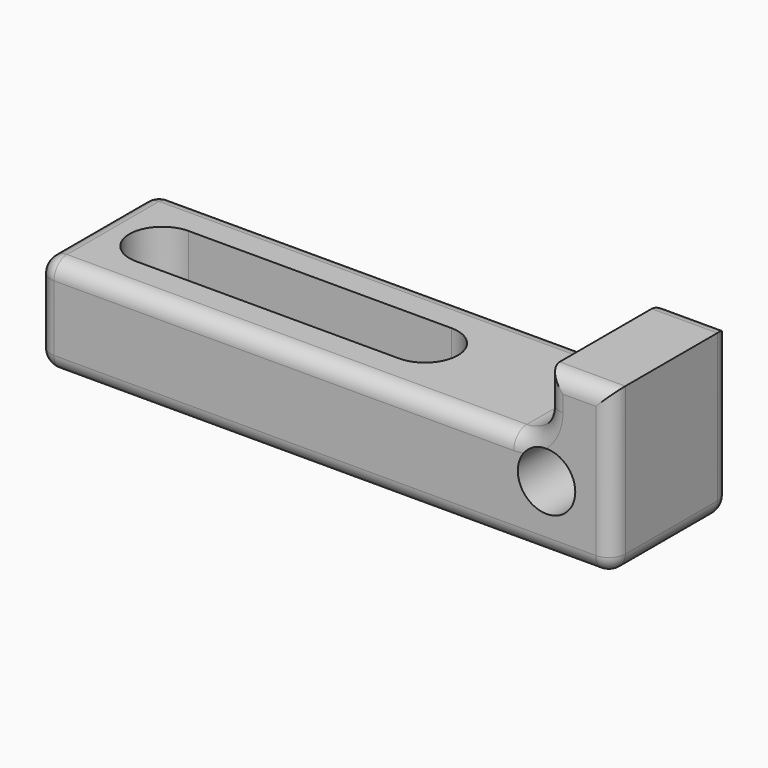
from build123d import *

# Parameters (mm, degrees)
F0_W         = 35
F0_H         = 9
F1_DEPTH     = 10
F2_R         = 1.75
F3_DEPTH     = 9.001
F5_DEPTH     = 6.001
F6_T1_DEPTH  = 28
F6_T3_DEPTH  = 7
F6_T5_DEPTH  = 9
F6_T7_DEPTH  = 33
F6_T9_DEPTH  = 4
F6_T11_DEPTH = 11.5
F6_T13_DEPTH = 4.5
F6_S17_W     = 1
F6_S17_H     = 1
F6_T18_DEPTH = 1
F6_S23_W     = 1
F6_S23_H     = 1
F6_T24_DEPTH = 1
F6_S29_W     = 1
F6_S29_H     = 1
F6_T30_DEPTH = 1
F6_S35_W     = 1
F6_S35_H     = 1
F6_T36_DEPTH = 1
F6_S41_W     = 1
F6_S41_H     = 1
F6_T42_DEPTH = 1
F6_S47_W     = 1
F6_S47_H     = 1
F6_T48_DEPTH = 1
F6_T52_ANGLE = 90
F6_T54_ANGLE = 90


# Not quite as in the source:
# - a fillet or chamfer that OpenCascade refuses, or shapes differently, is made with other operations: its cross-section is extruded or revolved along the edge and cut away or added


with BuildPart() as f1:
    # F0 (on Top) → F1 (new body)
    with BuildSketch(Plane.XY):
        Rectangle(F0_W, F0_H)
    extrude(amount=F1_DEPTH)

    # F2 (on face) → F3 (cut, through all)
    with BuildSketch(Plane.XZ.offset(4.5)):
        with BuildLine():
            Line((13.5, 10), (-17.5, 10))
            Line((-17.5, 10), (-17.5, 6))
            Line((-17.5, 6), (11.5, 6))
            ThreePointArc((11.5, 6), (12.9142135624, 6.5857864376), (13.5, 8))
            Line((13.5, 8), (13.5, 10))
        make_face()
        with Locations((13.5, 4)):
            Circle(F2_R)
    extrude(amount=-F3_DEPTH, mode=Mode.SUBTRACT)

    # F4 (on face) → F5 (cut, through all)
    with BuildSketch(Plane.XY.offset(6)):
        with BuildLine():
            ThreePointArc((-13.5, -2), (-12.0857864376, -1.4142135624), (-11.5, 0))
            ThreePointArc((-11.5, 0), (-12.0857864376, 1.4142135624), (-13.5, 2))
            ThreePointArc((-13.5, 2), (-15.5, 0), (-13.5, -2))
        make_face()
        with BuildLine():
            ThreePointArc((-13.5, 2), (-12.0857864376, 1.4142135624), (-11.5, 0))
            ThreePointArc((-11.5, 0), (-12.0857864376, -1.4142135624), (-13.5, -2))
            Line((-13.5, -2), (2.5, -2))
            ThreePointArc((2.5, -2), (0.5, 0), (2.5, 2))
            Line((2.5, 2), (-13.5, 2))
        make_face()
        with BuildLine():
            ThreePointArc((4.5, 0), (3.9142135624, 1.4142135624), (2.5, 2))
            ThreePointArc((2.5, 2), (0.5, 0), (2.5, -2))
            ThreePointArc((2.5, -2), (3.9142135624, -1.4142135624), (4.5, 0))
        make_face()
    extrude(amount=-F5_DEPTH, mode=Mode.SUBTRACT)

    # F6: fillet of radius 1 on 17 edges, made by hand

    # F6_s2 → F6_t1 (cut)
    with BuildSketch(Plane.YZ.offset(-16.5)):
        with BuildLine():
            ThreePointArc((-4.5, 5), (-4.2071067812, 5.7071067812), (-3.5, 6))
            Line((-3.5, 6), (-4.5, 6))
            Line((-4.5, 6), (-4.5, 5))
        make_face()
        with BuildLine():
            ThreePointArc((3.5, 6), (4.2071067812, 5.7071067812), (4.5, 5))
            Line((4.5, 5), (4.5, 6))
            Line((4.5, 6), (3.5, 6))
        make_face()
    extrude(amount=F6_T1_DEPTH, mode=Mode.SUBTRACT)

    # F6_s4 → F6_t3 (cut)
    with BuildSketch(Plane.XZ.offset(-3.5)):
        with BuildLine():
            ThreePointArc((-16.5, 6), (-17.2071067812, 5.7071067812), (-17.5, 5))
            Line((-17.5, 5), (-17.5, 6))
            Line((-17.5, 6), (-16.5, 6))
        make_face()
        with BuildLine():
            ThreePointArc((-16.5, 0), (-17.2071067812, 0.2928932188), (-17.5, 1))
            Line((-17.5, 1), (-17.5, 0))
            Line((-17.5, 0), (-16.5, 0))
        make_face()
        with BuildLine():
            ThreePointArc((16.5, 0), (17.2071067812, 0.2928932188), (17.5, 1))
            Line((17.5, 1), (17.5, 0))
            Line((17.5, 0), (16.5, 0))
        make_face()
    extrude(amount=F6_T3_DEPTH, mode=Mode.SUBTRACT)

    # F6_s6 → F6_t5 (cut)
    with BuildSketch(Plane.YZ.offset(11)):
        with BuildLine():
            ThreePointArc((-4.5, 9), (-4.2071067812, 9.7071067812), (-3.5, 10))
            Line((-3.5, 10), (-4.5, 10))
            Line((-4.5, 10), (-4.5, 9))
        make_face()
        with BuildLine():
            ThreePointArc((3.5, 10), (4.2071067812, 9.7071067812), (4.5, 9))
            Line((4.5, 9), (4.5, 10))
            Line((4.5, 10), (3.5, 10))
        make_face()
    extrude(amount=F6_T5_DEPTH, mode=Mode.SUBTRACT)

    # F6_s8 → F6_t7 (cut)
    with BuildSketch(Plane.YZ.offset(-16.5)):
        with BuildLine():
            ThreePointArc((-4.5, 1), (-4.2071067812, 0.2928932188), (-3.5, 0))
            Line((-3.5, 0), (-4.5, 0))
            Line((-4.5, 0), (-4.5, 1))
        make_face()
        with BuildLine():
            ThreePointArc((3.5, 0), (4.2071067812, 0.2928932188), (4.5, 1))
            Line((4.5, 1), (4.5, 0))
            Line((4.5, 0), (3.5, 0))
        make_face()
    extrude(amount=F6_T7_DEPTH, mode=Mode.SUBTRACT)

    # F6_s10 → F6_t9 (cut)
    with BuildSketch(Plane.XY.offset(1)):
        with BuildLine():
            ThreePointArc((-16.5, -4.5), (-17.2071067812, -4.2071067812), (-17.5, -3.5))
            Line((-17.5, -3.5), (-17.5, -4.5))
            Line((-17.5, -4.5), (-16.5, -4.5))
        make_face()
        with BuildLine():
            ThreePointArc((-17.5, 3.5), (-17.2071067812, 4.2071067812), (-16.5, 4.5))
            Line((-16.5, 4.5), (-17.5, 4.5))
            Line((-17.5, 4.5), (-17.5, 3.5))
        make_face()
    extrude(amount=F6_T9_DEPTH, mode=Mode.SUBTRACT)

    # F6_s12 → F6_t11 (cut)
    with BuildSketch(Plane.XY.offset(1)):
        with BuildLine():
            ThreePointArc((17.5, 3.5), (17.2071067812, 4.2071067812), (16.5, 4.5))
            Line((16.5, 4.5), (17.5, 4.5))
            Line((17.5, 4.5), (17.5, 3.5))
        make_face()
        with BuildLine():
            ThreePointArc((16.5, -4.5), (17.2071067812, -4.2071067812), (17.5, -3.5))
            Line((17.5, -3.5), (17.5, -4.5))
            Line((17.5, -4.5), (16.5, -4.5))
        make_face()
    extrude(amount=F6_T11_DEPTH, mode=Mode.SUBTRACT)

    # F6_s14 → F6_t13 (cut)
    with BuildSketch(Plane.XY.offset(8)):
        with BuildLine():
            ThreePointArc((14.5, -4.5), (13.7928932188, -4.2071067812), (13.5, -3.5))
            Line((13.5, -3.5), (13.5, -4.5))
            Line((13.5, -4.5), (14.5, -4.5))
        make_face()
        with BuildLine():
            ThreePointArc((13.5, 3.5), (13.7928932188, 4.2071067812), (14.5, 4.5))
            Line((14.5, 4.5), (13.5, 4.5))
            Line((13.5, 4.5), (13.5, 3.5))
        make_face()
    extrude(amount=F6_T13_DEPTH, mode=Mode.SUBTRACT)


with BuildPart() as f6_tool16:
    # F6_s17 → F6_t18 (new body)
    with BuildSketch(Plane.XZ.offset(3.5)):
        with Locations((-17, 5.5)):
            Rectangle(F6_S17_W, F6_S17_H)
    extrude(amount=F6_T18_DEPTH)

    # F6_s19 → F6_t20 (revolve, cut)
    with BuildSketch(Plane(origin=(-16.5, -3.5, 5), x_dir=(0.7071067812, 0, -0.7071067812), z_dir=(-0.7071067812, 0, -0.7071067812))):
        with BuildLine():
            ThreePointArc((0, -1), (1, 0), (0, 1))
            Line((0, 1), (0, -1))
        make_face()
    revolve(axis=Axis((-16.5, -3.5, 5), (0, -1, 0)), mode=Mode.SUBTRACT)


with BuildPart() as f1_1:
    add(f1.part)

    # F6_t15: cut F6_tool16
    add(f6_tool16.part, mode=Mode.SUBTRACT)


with BuildPart() as f6_tool22:
    # F6_s23 → F6_t24 (new body)
    with BuildSketch(Plane.XZ.offset(-3.5)):
        with Locations((-17, 5.5)):
            Rectangle(F6_S23_W, F6_S23_H)
    extrude(amount=-F6_T24_DEPTH)

    # F6_s25 → F6_t26 (revolve, cut)
    with BuildSketch(Plane(origin=(-16.5, 3.5, 5), x_dir=(0.7071067812, 0, -0.7071067812), z_dir=(0.7071067812, 0, 0.7071067812))):
        with BuildLine():
            ThreePointArc((0, -1), (1, 0), (0, 1))
            Line((0, 1), (0, -1))
        make_face()
    revolve(axis=Axis((-16.5, 3.5, 5), (0, 1, 0)), mode=Mode.SUBTRACT)


with BuildPart() as f1_2:
    add(f1_1.part)

    # F6_t21: cut F6_tool22
    add(f6_tool22.part, mode=Mode.SUBTRACT)


with BuildPart() as f6_tool28:
    # F6_s29 → F6_t30 (new body)
    with BuildSketch(Plane.XZ.offset(3.5)):
        with Locations((-17, 0.5)):
            Rectangle(F6_S29_W, F6_S29_H)
    extrude(amount=F6_T30_DEPTH)

    # F6_s31 → F6_t32 (revolve, cut)
    with BuildSketch(Plane(origin=(-16.5, -3.5, 1), x_dir=(0.7071067812, 0, 0.7071067812), z_dir=(0.7071067812, 0, -0.7071067812))):
        with BuildLine():
            ThreePointArc((0, -1), (1, 0), (0, 1))
            Line((0, 1), (0, -1))
        make_face()
    revolve(axis=Axis((-16.5, -3.5, 1), (0, -1, 0)), mode=Mode.SUBTRACT)


with BuildPart() as f1_3:
    add(f1_2.part)

    # F6_t27: cut F6_tool28
    add(f6_tool28.part, mode=Mode.SUBTRACT)


with BuildPart() as f6_tool34:
    # F6_s35 → F6_t36 (new body)
    with BuildSketch(Plane.XZ.offset(3.5)):
        with Locations((17, 0.5)):
            Rectangle(F6_S35_W, F6_S35_H)
    extrude(amount=F6_T36_DEPTH)

    # F6_s37 → F6_t38 (revolve, cut)
    with BuildSketch(Plane(origin=(16.5, -3.5, 1), x_dir=(-0.7071067812, 0, 0.7071067812), z_dir=(0.7071067812, 0, 0.7071067812))):
        with BuildLine():
            ThreePointArc((0, -1), (1, 0), (0, 1))
            Line((0, 1), (0, -1))
        make_face()
    revolve(axis=Axis((16.5, -3.5, 1), (0, -1, 0)), mode=Mode.SUBTRACT)


with BuildPart() as f1_4:
    add(f1_3.part)

    # F6_t33: cut F6_tool34
    add(f6_tool34.part, mode=Mode.SUBTRACT)


with BuildPart() as f6_tool40:
    # F6_s41 → F6_t42 (new body)
    with BuildSketch(Plane.XY.offset(1)):
        with Locations((-17, 4)):
            Rectangle(F6_S41_W, F6_S41_H)
    extrude(amount=-F6_T42_DEPTH)

    # F6_s43 → F6_t44 (revolve, cut)
    with BuildSketch(Plane(origin=(-16.5, 3.5, 1), x_dir=(0.7071067812, -0.7071067812, 0), z_dir=(0.7071067812, 0.7071067812, 0))):
        with BuildLine():
            ThreePointArc((0, -1), (1, 0), (0, 1))
            Line((0, 1), (0, -1))
        make_face()
    revolve(axis=Axis((-16.5, 3.5, 1), (0, 0, -1)), mode=Mode.SUBTRACT)


with BuildPart() as f1_5:
    add(f1_4.part)

    # F6_t39: cut F6_tool40
    add(f6_tool40.part, mode=Mode.SUBTRACT)


with BuildPart() as f6_tool46:
    # F6_s47 → F6_t48 (new body)
    with BuildSketch(Plane.XY.offset(1)):
        with Locations((17, 4)):
            Rectangle(F6_S47_W, F6_S47_H)
    extrude(amount=-F6_T48_DEPTH)

    # F6_s49 → F6_t50 (revolve, cut)
    with BuildSketch(Plane(origin=(16.5, 3.5, 1), x_dir=(-0.7071067812, -0.7071067812, 0), z_dir=(0.7071067812, -0.7071067812, 0))):
        with BuildLine():
            ThreePointArc((0, -1), (1, 0), (0, 1))
            Line((0, 1), (0, -1))
        make_face()
    revolve(axis=Axis((16.5, 3.5, 1), (0, 0, -1)), mode=Mode.SUBTRACT)


with BuildPart() as f1_6:
    add(f1_5.part)

    # F6_t45: cut F6_tool46
    add(f6_tool46.part, mode=Mode.SUBTRACT)

    # F6_s51 → F6_t52 (revolve, cut)
    with BuildSketch(Plane.YZ.offset(11.5)):
        with BuildLine():
            ThreePointArc((-4.5, 5), (-4.2071067812, 5.7071067812), (-3.5, 6))
            Line((-3.5, 6), (-4.5, 6))
            Line((-4.5, 6), (-4.5, 5))
        make_face()
    revolve(axis=Axis((11.5, -4.5, 8), (0, -1, 0)), revolution_arc=F6_T52_ANGLE, mode=Mode.SUBTRACT)

    # F6_s53 → F6_t54 (revolve, cut)
    with BuildSketch(Plane.YZ.offset(11.5)):
        with BuildLine():
            ThreePointArc((3.5, 6), (4.2071067812, 5.7071067812), (4.5, 5))
            Line((4.5, 5), (4.5, 6))
            Line((4.5, 6), (3.5, 6))
        make_face()
    revolve(axis=Axis((11.5, 4.5, 8), (0, -1, 0)), revolution_arc=F6_T54_ANGLE, mode=Mode.SUBTRACT)


solid = f1_6.part
